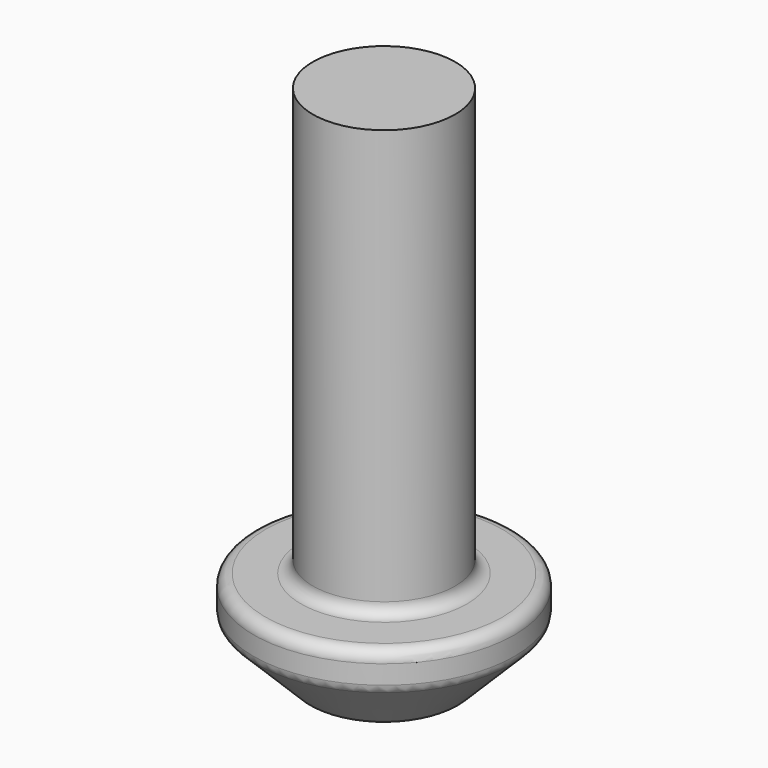
from build123d import *

# Parameters (mm, degrees)
F1_R     = 2.75
F1_R_2   = 1.5
F2_DEPTH = 2
F3_START = 1.5
F3_DEPTH = 0.5
F4_START = 2
F4_DEPTH = 9
F5_SIZE2 = 1.25
F5_SIZE  = 1.25
F6_R     = 0.25


# Not quite as in the source:
# - a feature names something its author has since deleted; it is built from what else it names


with BuildPart() as f2:
    # F1 (on Top) → F2 (new body)
    with BuildSketch(Plane.XY):
        Circle(F1_R)
        Circle(F1_R_2, mode=Mode.SUBTRACT)
        Circle(F1_R_2)
        Polygon((-0.5773502692, -1), (-1.1547005384, 0), (-0.5773502692, 1), (0.5773502692, 1), (1.1547005384, 0), (0.5773502692, -1), align=None, mode=Mode.SUBTRACT)
    extrude(amount=F2_DEPTH)

    # F1 (on Top) → F3 (join)
    with BuildSketch(Plane.XY.offset(F3_START)):
        Polygon((-0.5773502692, 1), (-1.1547005384, 0), (-0.5773502692, -1), (0.5773502692, -1), (1.1547005384, 0), (0.5773502692, 1), align=None)
    extrude(amount=F3_DEPTH)

    # F1 (on Top) → F4 (join)
    with BuildSketch(Plane.XY.offset(F4_START)):
        Circle(F1_R_2)
        Polygon((-0.5773502692, -1), (-1.1547005384, 0), (-0.5773502692, 1), (0.5773502692, 1), (1.1547005384, 0), (0.5773502692, -1), align=None, mode=Mode.SUBTRACT)
        Polygon((-0.5773502692, 1), (-1.1547005384, 0), (-0.5773502692, -1), (0.5773502692, -1), (1.1547005384, 0), (0.5773502692, 1), align=None)
    extrude(amount=F4_DEPTH)

    # F5
    f5_edges = [f2.edges().sort_by_distance(p)[0] for p in [
        (-2.75, 0, 0),
    ]]
    chamfer(f5_edges, length=F5_SIZE, length2=F5_SIZE2)

    # F6
    f6_edges = [f2.edges().sort_by_distance(p)[0] for p in [
        (-2.75, 0, 2),
        (-1.5, 0, 2),
        (-1.5, 0, 0),
        (-2.75, 0, 1.25),
    ]]
    fillet(f6_edges, radius=F6_R)


solid = f2.part
